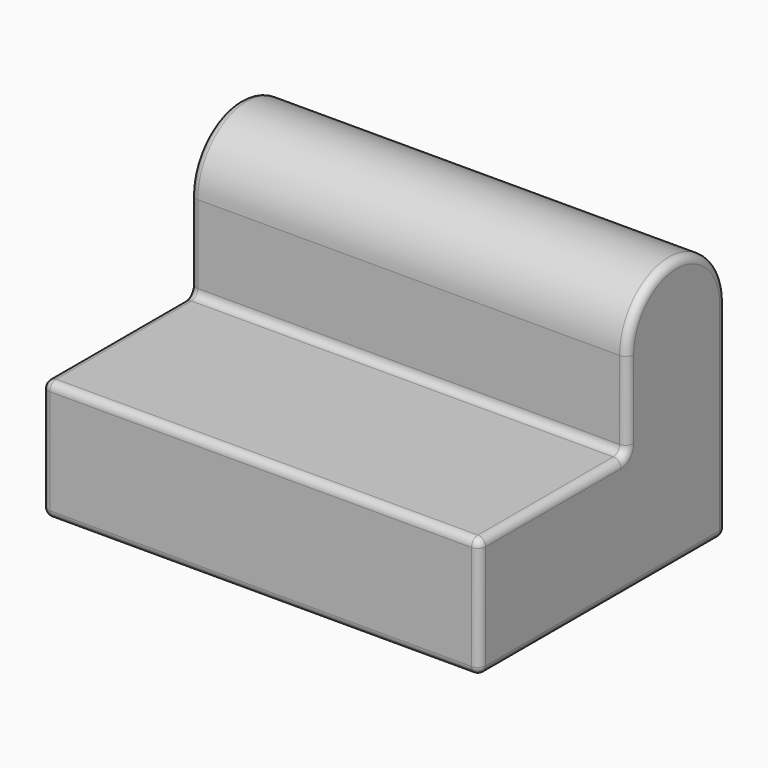
from build123d import *

# Parameters (mm, degrees)
F1_DEPTH = 709.6125
F2_R     = 25.4
F3_SCALE = 0.05


with BuildPart() as f1:
    # F0 (on Right) → F1 (new body, symmetric)
    with BuildSketch(Plane.YZ):
        with BuildLine():
            Line((-1000.125, 0), (0, 0))
            Line((0, 0), (0, 669.925))
            ThreePointArc((0, 669.925), (-200.025, 869.95), (-400.05, 669.925))
            Line((-400.05, 669.925), (-400.05, 390.525))
            Line((-400.05, 390.525), (-1000.125, 390.525))
            Line((-1000.125, 390.525), (-1000.125, 0))
        make_face()
    extrude(amount=F1_DEPTH, both=True)

    # F2
    f2_edges = [f1.edges().sort_by_distance(p)[0] for p in [
        (709.6125, 0, 334.9625),
        (-709.6125, -500.0625, 0),
        (0, 0, 0),
        (709.6125, -500.0625, 0),
        (0, -1000.125, 0),
        (-709.6125, 0, 334.9625),
        (-709.6125, -200.025, 869.95),
        (-709.6125, -400.05, 530.225),
        (-709.6125, -700.0875, 390.525),
        (-709.6125, -1000.125, 195.2625),
        (0, -1000.125, 390.525),
        (709.6125, -200.025, 869.95),
        (709.6125, -400.05, 530.225),
        (709.6125, -700.0875, 390.525),
        (709.6125, -1000.125, 195.2625),
        (0, -400.05, 390.525),
        (0, -400.05, 669.925),
        (0, 0, 669.925),
    ]]
    fillet(f2_edges, radius=F2_R)


with BuildPart() as f1_1:
    # F3: moved
    add(f1.part.scale(F3_SCALE))


solid = f1_1.part
